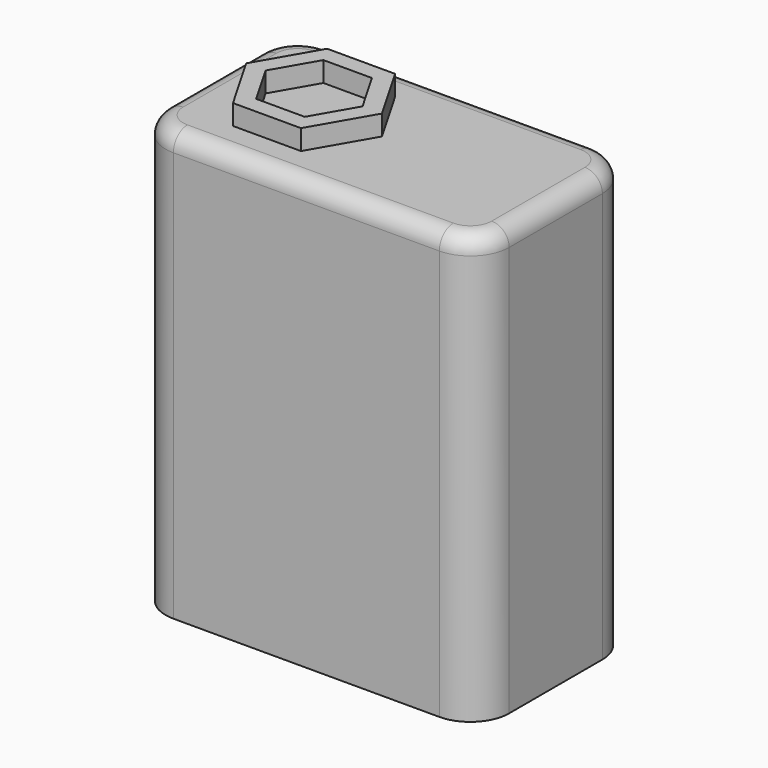
from build123d import *

# Parameters (mm, degrees)
F0_W     = 44.9535958469
F0_H     = 55.96075207
F1_DEPTH = 25.4
F2_R     = 5.08
F7_DEPTH = 2.6416
F8_R     = 2.286


# Not quite as in the source:
# - the program builds the solid bodies; features that only make, move or delete a surface that nothing else refers to are left out


with BuildPart() as f1:
    # F0 (on Front) → F1 (new body)
    with BuildSketch(Plane.XZ):
        with Locations((-22.4767979234, 27.980376035)):
            Rectangle(F0_W, F0_H)
    extrude(amount=F1_DEPTH)

    # F2
    f2_edges = [f1.edges().sort_by_distance(p)[0] for p in [
        (-44.953596, -25.4, 27.980376),
        (-44.953596, 0, 27.980376),
        (0, -25.4, 27.980376),
        (0, 0, 27.980376),
    ]]
    fillet(f2_edges, radius=F2_R)

    # F6 (on face) → F7 (join)
    with BuildSketch(Plane.XY.offset(55.96075207)):
        Polygon((-36.077086072, -5.0010341604), (-40.522086072, -12.7), (-36.077086072, -20.3989658396), (-27.187086072, -20.3989658396), (-22.742086072, -12.7), (-27.187086072, -5.0010341604), align=None)
        Polygon((-34.807086072, -18.199261314), (-37.982086072, -12.7), (-34.807086072, -7.200738686), (-28.457086072, -7.200738686), (-25.282086072, -12.7), (-28.457086072, -18.199261314), align=None, mode=Mode.SUBTRACT)
    extrude(amount=F7_DEPTH)

    # F8
    f8_edges = [f1.edges().sort_by_distance(p)[0] for p in [
        (-22.476798, -25.4, 55.960752),
    ]]
    fillet(f8_edges, radius=F8_R)


solid = f1.part
